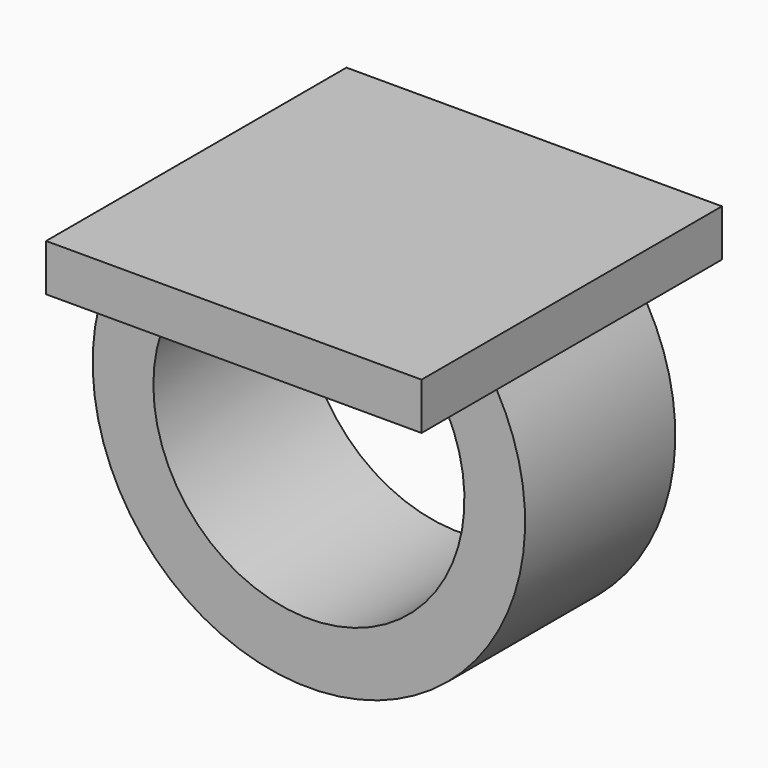
from build123d import *
from build123d import SkipClean  # not in build123d's __all__

# Parameters (mm, degrees)
F0_W          = 25.4
F0_H          = 25.4
F1_DEPTH      = 3.175
F3_W          = 5.08
F3_H          = 12.7
F6_DEPTH      = 6.35
F6_DEPTH_BACK = 6.35


with BuildPart() as f1:
    # F0 (on Top) → F1 (new body)
    with BuildSketch(Plane.XY):
        Rectangle(F0_W, F0_H)
    extrude(amount=F1_DEPTH)

    # F4: sweep along a path in F2
    with BuildLine(Plane.XZ) as f4_path:
        ThreePointArc((-10.16, 0), (0, -19.7423783289), (10.16, 0))
    # F3 (on face) → F4 (sweep)
    with BuildSketch(Plane(origin=(0, 0, 0), x_dir=(1, 0, 0), z_dir=(0, 0, -1))):
        with Locations((-10.16, 0)):
            Rectangle(F3_W, F3_H)
    sweep(path=f4_path.line)

    # F5 (on Front) → F6 (join, two sides)
    with BuildSketch(Plane.XZ) as f6_sk:
        with BuildLine():
            Line((9.3361319986, -2.4026738264), (10.16, 0))
            Line((10.16, 0), (7.62, 0))
            ThreePointArc((7.62, 0), (8.5627573519, -1.1408453315), (9.3361319986, -2.4026738264))
        make_face()
    with SkipClean():  # cleaning this boolean's faces spoils the solid; the shape is the same uncleaned
        extrude(amount=F6_DEPTH)
        extrude(f6_sk.sketch, amount=-F6_DEPTH_BACK)


solid = f1.part
